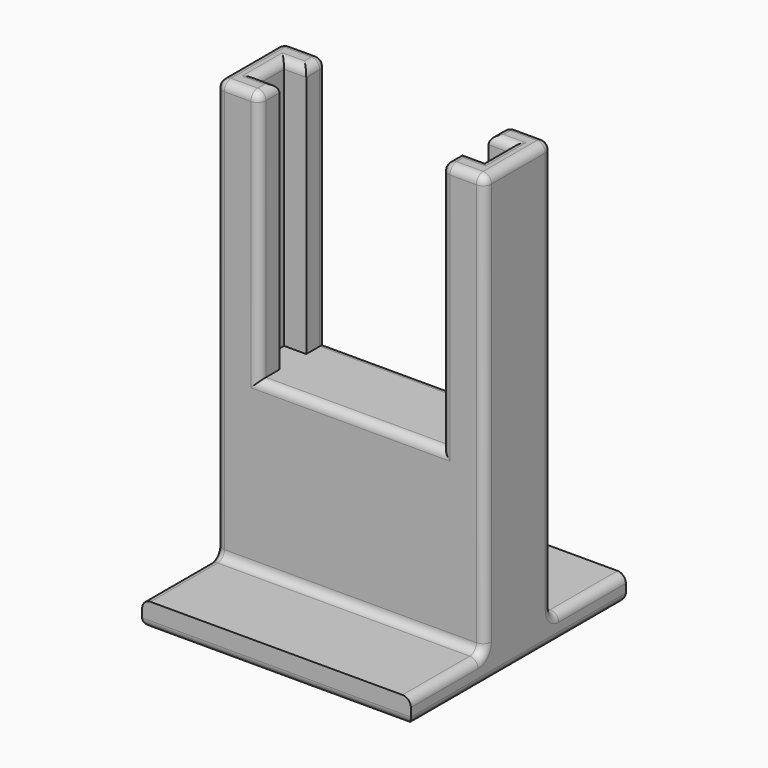
from build123d import *

# Parameters (mm, degrees)
F0_W     = 32
F0_H     = 32
F1_DEPTH = 3
F2_W     = 32
F2_H     = 10
F3_DEPTH = 50
F5_DEPTH = 30
F6_F1_R  = 1
F6_F2_R  = 1


with BuildPart() as f1:
    # F0 (on Top) → F1 (new body)
    with BuildSketch(Plane.XY):
        Rectangle(F0_W, F0_H)
    extrude(amount=F1_DEPTH)

    # F2 (on face) → F3 (join)
    with BuildSketch(Plane.XY.offset(3)):
        Rectangle(F2_W, F2_H)
    extrude(amount=F3_DEPTH)

    # F4 (on face) → F5 (cut)
    with BuildSketch(Plane.XY.offset(53)):
        Polygon((10.8576942235, 5), (-10.8576942235, 5), (-10.8576942235, 2), (-13.5, 2), (-13.5, -2), (-10.8576942235, -2), (-10.8576942235, -5), (10.8576942235, -5), (10.8576942235, -2), (13.5, -2), (13.5, 2), (10.8576942235, 2), align=None)
    extrude(amount=-F5_DEPTH, mode=Mode.SUBTRACT)

    # F6: fillet of radius 1 on 32 edges, made by hand

    # F6_f1
    f6_f1_edges = [f1.edges().sort_by_distance(p)[0] for p in [
        (0, -5, 3),
        (0, 5, 3),
    ]]
    fillet(f6_f1_edges, radius=F6_F1_R)

    # F6_f2
    f6_f2_edges = [f1.edges().sort_by_distance(p)[0] for p in [
        (0, 16, 0),
        (-16, 0, 0),
        (0, -16, 0),
        (16, 0, 0),
        (16, -5, 28.5),
        (13.4288471118, -5, 53),
        (10.8576942235, -5, 38),
        (0, -5, 23),
        (-10.8576942235, -5, 38),
        (-13.4288471118, -5, 53),
        (-16, -5, 28.5),
        (-16, 5, 28.5),
        (-13.4288471118, 5, 53),
        (-10.8576942235, 5, 38),
        (0, 5, 23),
        (10.8576942235, 5, 38),
        (13.4288471118, 5, 53),
        (16, 5, 28.5),
        (16, 0, 53),
        (10.8576942235, -3.5, 53),
        (12.1788471118, -2, 53),
        (13.5, 0, 53),
        (12.1788471118, 2, 53),
        (10.8576942235, 3.5, 53),
        (-10.8576942235, 3.5, 53),
        (-12.1788471118, 2, 53),
        (-13.5, 0, 53),
        (-12.1788471118, -2, 53),
        (-10.8576942235, -3.5, 53),
        (-16, 0, 53),
        (16, 5.2928932188, 3.2928932188),
        (-16, 5.2928932188, 3.2928932188),
        (-16, -5.2928932188, 3.2928932188),
        (16, -5.2928932188, 3.2928932188),
    ]]
    fillet(f6_f2_edges, radius=F6_F2_R)


solid = f1.part
